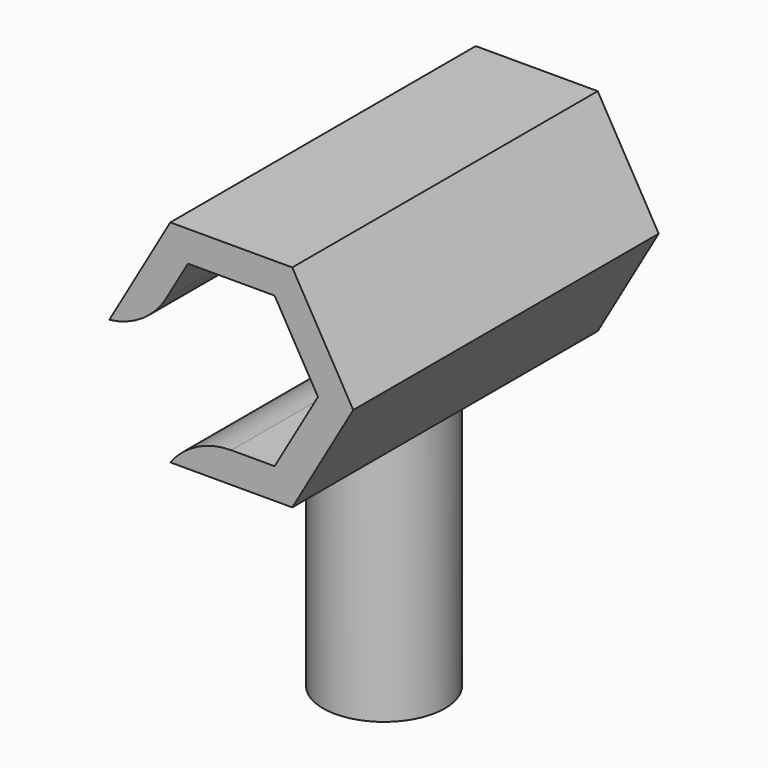
from build123d import *

# Parameters (mm, degrees)
F1_DEPTH    = 15
F2_T1_DEPTH = 23.5358983849
F3_R        = 1.5
F4_DEPTH    = 10


# Not quite as in the source:
# - a fillet or chamfer that OpenCascade refuses, or shapes differently, is made with other operations: its cross-section is extruded or revolved along the edge and cut away or added


with BuildPart() as f1:
    # F0 (on Front) → F1 (new body)
    with BuildSketch(Plane.XZ):
        Polygon((-3.4063665882, 0), (-1.7031832941, 2.95), (1.7031832941, 2.95), (3.4063665882, 0), (1.7031832941, -2.95), (-1.7031832941, -2.95), (-2.3960036171, -4.15), (2.3960036171, -4.15), (4.7920072343, 0), (2.3960036171, 4.15), (-2.3960036171, 4.15), (-4.7920072343, 0), align=None)
    extrude(amount=F1_DEPTH)

    # F2: fillet of radius 3 on 2 edges, made by hand

    # F2_s2 → F2_t1 (cut)
    with BuildSketch(Plane.XZ.offset(-4.2679491924)):
        with BuildLine():
            ThreePointArc((-4.7920072343, 0), (-3.4978833466, 0.4749251787), (-2.5527767497, 1.4784609691))
            Line((-2.5527767497, 1.4784609691), (-3.4063665882, 0))
            Line((-3.4063665882, 0), (-4.7920072343, 0))
        make_face()
        with BuildLine():
            ThreePointArc((0.0039963829, -2.95), (-1.3376444036, -3.266718427), (-2.3960036171, -4.15))
            Line((-2.3960036171, -4.15), (-1.7031832941, -2.95))
            Line((-1.7031832941, -2.95), (0.0039963829, -2.95))
        make_face()
    extrude(amount=F2_T1_DEPTH, mode=Mode.SUBTRACT)

    # F3 (on face) → F4 (join)
    with BuildSketch(Plane(origin=(0, 0, -4.15), x_dir=(1, 0, 0), z_dir=(0, 0, -1))):
        with BuildLine():
            ThreePointArc((-2.3960036171, 7.5), (0, 5.1039963829), (2.3960036171, 7.5))
            ThreePointArc((2.3960036171, 7.5), (0, 9.8960036171), (-2.3960036171, 7.5))
        make_face()
        with Locations((0, 7.5)):
            Circle(F3_R, mode=Mode.SUBTRACT)
    extrude(amount=F4_DEPTH)


solid = f1.part
